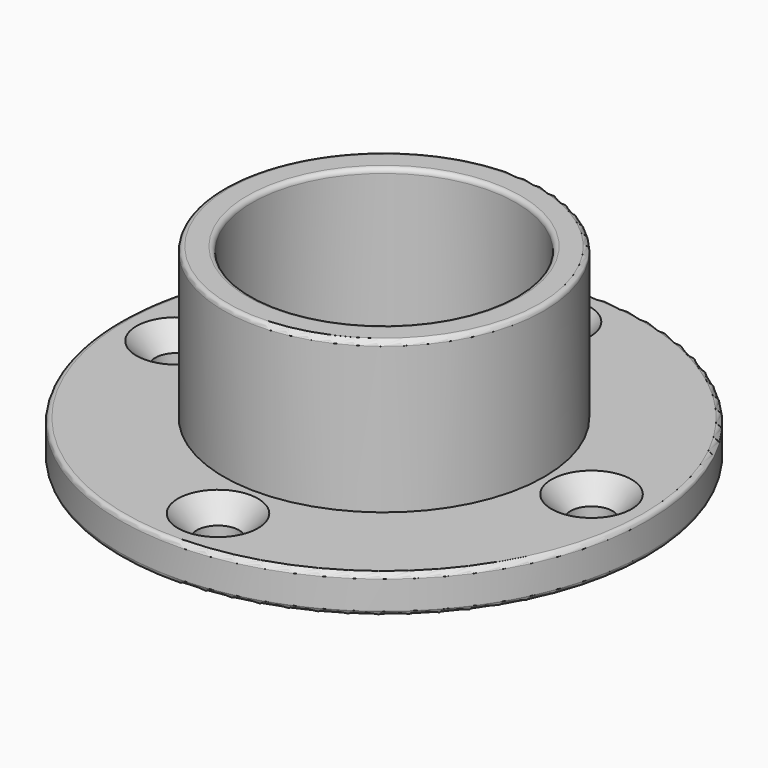
from build123d import *

# Parameters (mm, degrees)
F0_R           = 26.9875
F0_R_2         = 22.225
F1_DEPTH       = 25.4
F0_R_3         = 44.45
F1_FACE_R      = 26.9875
F1_FACE_R_2    = 22.225
F2_DEPTH       = 6.35
F4_D           = 7.1374
F4_CSINK_D     = 13.4874
F4_CSINK_ANGLE = 82
F5_R           = 0.79375


with BuildPart() as f1:
    # F0 (on Top) → F1 (new body)
    with BuildSketch(Plane.XY):
        Circle(F0_R)
        Circle(F0_R_2, mode=Mode.SUBTRACT)
    extrude(amount=F1_DEPTH)

    # F0 (on Top) + F1_face (on face) → F2 (join)
    with BuildSketch(Plane.XY):
        Circle(F0_R_3)
        Circle(F0_R, mode=Mode.SUBTRACT)
        Circle(F0_R)
        Circle(F0_R_2, mode=Mode.SUBTRACT)
        Circle(F0_R_2)
    with BuildSketch(Plane(origin=(0, 0, 0), x_dir=(1, 0, 0), z_dir=(0, 0, -1))):
        Circle(F1_FACE_R)
        Circle(F1_FACE_R_2, mode=Mode.SUBTRACT)
    extrude(amount=-F2_DEPTH, dir=(0, 0, 1))

    # F4 (through all)
    with Locations(Plane.XY):
        with Locations((-34.925, 0), (0, 34.925), (34.925, 0), (0, -34.925)):
            CounterSinkHole(F4_D / 2, F4_CSINK_D / 2, counter_sink_angle=F4_CSINK_ANGLE)

    # F5
    f5_edges = [f1.edges().sort_by_distance(p)[0] for p in [
        (-26.9875, 0, 25.4),
        (-44.45, 0, 0),
        (-44.45, 0, -6.35),
        (-3.5687, -34.925, -6.35),
        (-38.4937, 0, -6.35),
        (31.3563, 0, -6.35),
        (-3.5687, 34.925, -6.35),
        (-22.225, 0, 25.4),
        (22.225, 0, 12.7),
        (-22.225, 0, 0),
    ]]
    fillet(f5_edges, radius=F5_R)


solid = f1.part
